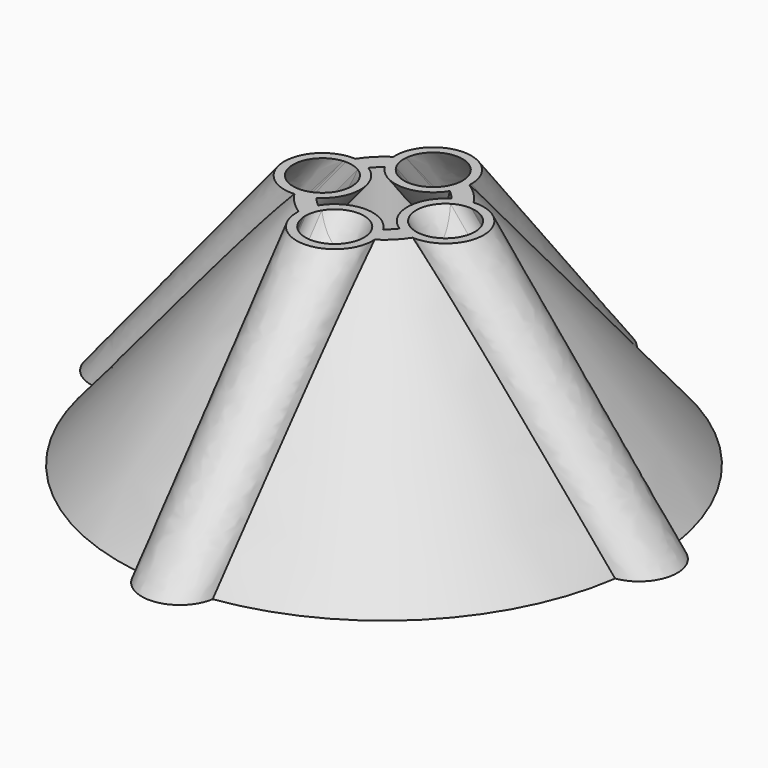
from build123d import *

# Parameters (mm, degrees)
F7_COUNT = 4
F8_COUNT = 4


with BuildPart() as f1:
    # F0 (on Front) → F1 (revolve)
    with BuildSketch(Plane.XZ):
        Polygon((-0.9, 0), (-0.9, 4), (-1.2, 4), (-4.5, 0), align=None)
    revolve(axis=Axis((0, 0, 2), (0, 0, 1)))

    # F5: sweep along a path in F4
    with BuildLine(Plane(origin=(0, 0, 0), x_dir=(0, -1, 0), z_dir=(-1, 0, 0))) as f5_path:
        Line((-4.5, 0), (-1.2, 4))
    # F2 (on face) → F5 (sweep)
    with BuildSketch(Plane.XY.offset(4)):
        with BuildLine():
            ThreePointArc((0.6487385282, 1.0095238095), (0.6496845555, 1.0297520785), (0.65, 1.05))
            ThreePointArc((0.65, 1.05), (-0.0202479215, 1.6996845555), (-0.6487385282, 1.0095238095))
            ThreePointArc((-0.6487385282, 1.0095238095), (-0.5749684894, 1.0532859233), (-0.4982608643, 1.0916666667))
            ThreePointArc((-0.4982608643, 1.0916666667), (0, 1.55), (0.4982608643, 1.0916666667))
            ThreePointArc((0.4982608643, 1.0916666667), (0.5749684894, 1.0532859233), (0.6487385282, 1.0095238095))
        make_face()
        with BuildLine():
            ThreePointArc((-0.4982608643, 1.0916666667), (-0.5749684894, 1.0532859233), (-0.6487385282, 1.0095238095))
            ThreePointArc((-0.6487385282, 1.0095238095), (-0.6196453896, 0.8536849696), (-0.553693023, 0.7095238095))
            ThreePointArc((-0.553693023, 0.7095238095), (-0.4926083303, 0.7532177859), (-0.428093318, 0.7916666667))
            ThreePointArc((-0.428093318, 0.7916666667), (-0.4868603678, 0.936127342), (-0.4982608643, 1.0916666667))
        make_face()
        with BuildLine():
            ThreePointArc((-0.428093318, 0.7916666667), (-0.4926083303, 0.7532177859), (-0.553693023, 0.7095238095))
            ThreePointArc((-0.553693023, 0.7095238095), (0, 0.4), (0.553693023, 0.7095238095))
            ThreePointArc((0.553693023, 0.7095238095), (0.4926083303, 0.7532177859), (0.428093318, 0.7916666667))
            ThreePointArc((0.428093318, 0.7916666667), (0, 0.55), (-0.428093318, 0.7916666667))
        make_face()
        with BuildLine():
            ThreePointArc((0.553693023, 0.7095238095), (0.6196453896, 0.8536849696), (0.6487385282, 1.0095238095))
            ThreePointArc((0.6487385282, 1.0095238095), (0.5749684894, 1.0532859233), (0.4982608643, 1.0916666667))
            ThreePointArc((0.4982608643, 1.0916666667), (0.4995650269, 1.070851473), (0.5, 1.05))
            ThreePointArc((0.5, 1.05), (0.4816880002, 0.9159228934), (0.428093318, 0.7916666667))
            ThreePointArc((0.428093318, 0.7916666667), (0.4926083303, 0.7532177859), (0.553693023, 0.7095238095))
        make_face()
    sweep(path=f5_path.line)

    # F6: sweep along a path in F4
    with BuildLine(Plane(origin=(0, 0, 0), x_dir=(0, -1, 0), z_dir=(-1, 0, 0))) as f6_path:
        Line((-4.5, 0), (-1.2, 4))
    # F2 (on face) → F6 (sweep, cut)
    with BuildSketch(Plane.XY.offset(4)):
        with BuildLine():
            ThreePointArc((0.4982608643, 1.0916666667), (0, 1.55), (-0.4982608643, 1.0916666667))
            ThreePointArc((-0.4982608643, 1.0916666667), (0, 1.2), (0.4982608643, 1.0916666667))
        make_face()
        with BuildLine():
            ThreePointArc((0.428093318, 0.7916666667), (0, 0.9), (-0.428093318, 0.7916666667))
            ThreePointArc((-0.428093318, 0.7916666667), (0, 0.55), (0.428093318, 0.7916666667))
        make_face()
        with BuildLine():
            ThreePointArc((0.4982608643, 1.0916666667), (0, 1.2), (-0.4982608643, 1.0916666667))
            ThreePointArc((-0.4982608643, 1.0916666667), (-0.4868603678, 0.936127342), (-0.428093318, 0.7916666667))
            ThreePointArc((-0.428093318, 0.7916666667), (0, 0.9), (0.428093318, 0.7916666667))
            ThreePointArc((0.428093318, 0.7916666667), (0.4816880002, 0.9159228934), (0.5, 1.05))
            ThreePointArc((0.5, 1.05), (0.4995650269, 1.070851473), (0.4982608643, 1.0916666667))
        make_face()
    f6 = sweep(path=f6_path.line, mode=Mode.SUBTRACT)

    # F7: F6 ×4 about axis
    f7_axis = Axis((0, 0, 4), (0, 0, -1))
    for i in range(1, F7_COUNT):
        add(f6.rotate(f7_axis, i * 360 / F7_COUNT), mode=Mode.SUBTRACT)


with BuildPart() as f8_1:
    # F8: instance of F1
    add(f1.part.rotate(Axis((0, 0, 0), (0, 0, 1)), 1 * 360 / F8_COUNT))


with BuildPart() as f8_2:
    # F8: instance of F1
    add(f1.part.rotate(Axis((0, 0, 0), (0, 0, 1)), 2 * 360 / F8_COUNT))


with BuildPart() as f8_3:
    # F8: instance of F1
    add(f1.part.rotate(Axis((0, 0, 0), (0, 0, 1)), 3 * 360 / F8_COUNT))


with BuildPart() as f8_2_1:
    add(f8_2.part)

    # F9: union F8_3, F1, F8_1
    add(f8_3.part)
    add(f1.part)
    add(f8_1.part)


solid = f8_2_1.part
